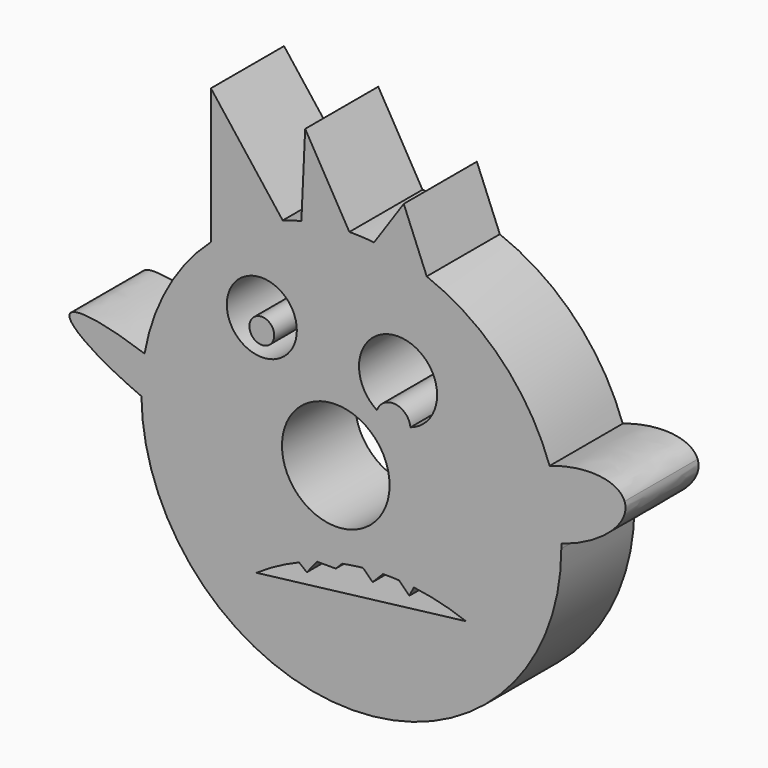
from build123d import *

# Parameters (mm, degrees)
F0_R     = 14.9564951484
F0_R_2   = 9.7335574138
F1_DEPTH = 25.4
F0_R_3   = 3.456724349


# Not quite as in the source:
# - a feature names something its author has since deleted; it is built from what else it names
# - the program builds the solid bodies; features that only make, move or delete a surface that nothing else refers to are left out


with BuildPart() as f1:
    # F0 (on Front) → F1 (new body)
    with BuildSketch(Plane.XZ):
        with BuildLine():
            Line((29.2069212967, 44.8178982187), (-33.0534157144, 44.8178982187))
            ThreePointArc((-33.0534157144, 44.8178982187), (-33.8848589906, 44.1111281894), (-34.7029421619, 43.3889358876))
            ThreePointArc((-34.7029421619, 43.3889358876), (-46.7244943553, 28.2782026704), (-53.157396148, 10.0718919506))
            add(Edge.make_bspline(
                [(-54.0295326022, -0.6419861495), (-25.6291677814, -12.7776607333), (-25.1074200255, -6.368179936), (-24.5856722696, 0.0413008612), (-53.157396148, 10.0718919506)],
                knots=[1.4674967071, 1.4674967071, 1.4674967071, 3.2032565901, 3.2032565901, 4.9390164731, 4.9390164731, 4.9390164731], degree=2, weights=[1, 0.646445519, 1, 0.646445519, 1]))
            ThreePointArc((-54.0295326022, -0.6419861495), (4.6490094653, -58.3601924627), (62.6890867818, 0))
            ThreePointArc((62.6890867818, 0), (62.6859343797, 0.6065848839), (62.6764775138, 1.2131042379))
            add(Edge.make_bspline(
                [(59.4330403873, 19.2211055653), (41.4698148053, 12.9716188145), (43.0336953944, 4.2887424007), (44.5975759835, -4.3941340131), (62.6764775138, 1.2131042379)],
                knots=[1.5260344916, 1.5260344916, 1.5260344916, 3.0598387567, 3.0598387567, 4.5936430218, 4.5936430218, 4.5936430218], degree=2, weights=[1, 0.720063756, 1, 0.720063756, 1]))
            ThreePointArc((59.4330403873, 19.2211055653), (46.2413654037, 40.611400757), (25.2778493531, 54.4712713212))
            Line((25.2778493531, 54.4712713212), (29.2069212967, 44.8178982187))
        make_face()
        Circle(F0_R, mode=Mode.SUBTRACT)
        with BuildLine():
            ThreePointArc((21.6792569731, -22.7834417511), (29.0444233173, -24.1430496826), (36.1979231238, -26.361528784))
            Line((36.1979231238, -26.361528784), (-22.0335181803, -33.4437340498))
            ThreePointArc((-22.0335181803, -33.4437340498), (-16.2921483285, -29.9333256583), (-10.2111068854, -27.0510991203))
            Line((-10.2111068854, -27.0510991204), (-14.6030960605, -23.5375072807))
            Line((-14.6030960605, -23.5375072807), (5.047085695, -20.1314762235))
            Line((5.047085695, -20.1314762235), (24.1732671857, -17.7734531462))
            Line((24.1732671857, -17.7734531462), (21.6792569731, -22.7834417511))
        make_face(mode=Mode.SUBTRACT)
        with Locations((-20.5633433886, 29.5139586047)):
            Circle(F0_R_2, mode=Mode.SUBTRACT)
        with BuildLine():
            ThreePointArc((11.440167814, 17.2330375959), (12.1122768861, 35.8889061597), (28.1660100748, 26.361534372))
            ThreePointArc((28.1660100748, 26.361534372), (26.117377722, 20.0153029261), (20.7448195069, 16.0647122986))
            ThreePointArc((20.7448195069, 16.0647122986), (20.7622755027, 15.8287118822), (20.7680988698, 15.5921384334))
            ThreePointArc((20.7680988698, 15.5921384334), (15.1267587025, 10.8565590643), (11.440167814, 17.2330375959))
        make_face(mode=Mode.SUBTRACT)
        with BuildLine():
            ThreePointArc((-14.7525066988, 55.1538659378), (-24.3720908883, 50.8165251157), (-33.0534157144, 44.8178982187))
            Line((-33.0534157144, 44.8178982187), (29.2069212967, 44.8178982187))
            Line((29.2069212967, 44.8178982187), (25.2778493531, 54.4712713212))
            ThreePointArc((25.2778493531, 54.4712713212), (18.0685855983, 56.7204701), (10.6292413524, 58.0199069867))
            Line((10.6292413524, 58.0199069867), (7.0293885895, 52.7346457751))
            Line((7.0293885895, 52.7346457751), (3.7755604577, 58.3584604129))
            ThreePointArc((3.7755604577, 58.3584604129), (-2.9439825789, 57.9062449617), (-9.5666869161, 56.6829115246))
            Line((-9.5666869161, 56.6829115246), (-9.9255512055, 48.9001048884))
            Line((-9.9255512055, 48.9001048884), (-14.7525066988, 55.1538659378))
        make_face()
        with BuildLine():
            ThreePointArc((-34.7029421619, 43.3889358876), (-33.8848589906, 44.1111281894), (-33.0534157144, 44.8178982187))
            ThreePointArc((-33.0534157144, 44.8178982187), (-24.3720908883, 50.8165251157), (-14.7525066988, 55.1538659378))
            Line((-14.7525066988, 55.1538659378), (-34.7029421619, 81.0014745162))
            Line((-34.7029421619, 81.0014745162), (-34.7029421619, 43.3889358876))
        make_face()
        with BuildLine():
            add(Edge.make_bspline(
                [(80.264955759, 17.3160471022), (77.2571204557, 25.4221829679), (59.4330403873, 19.2211055653)],
                knots=[0, 0, 0, 1.5260344916, 1.5260344916, 1.5260344916], degree=2, weights=[1, 0.7227540692, 1]))
            ThreePointArc((59.4330403873, 19.2211055653), (61.7648977694, 10.3450086355), (62.6764775138, 1.2131042379))
            add(Edge.make_bspline(
                [(62.6764775138, 1.2131042379), (83.8081315933, 7.7671649955), (80.264955759, 17.3160471022)],
                knots=[4.5936430218, 4.5936430218, 4.5936430218, 6.2831853072, 6.2831853072, 6.2831853072], degree=2, weights=[1, 0.6639024438, 1]))
        make_face()
        with BuildLine():
            ThreePointArc((62.6764775138, 1.2131042379), (61.7648977694, 10.3450086355), (59.4330403873, 19.2211055653))
            add(Edge.make_bspline(
                [(59.4330403873, 19.2211055653), (41.4698148053, 12.9716188145), (43.0336953944, 4.2887424007), (44.5975759835, -4.3941340131), (62.6764775138, 1.2131042379)],
                knots=[1.5260344916, 1.5260344916, 1.5260344916, 3.0598387567, 3.0598387567, 4.5936430218, 4.5936430218, 4.5936430218], degree=2, weights=[1, 0.720063756, 1, 0.720063756, 1]))
        make_face()
        with BuildLine():
            add(Edge.make_bspline(
                [(-54.0295326022, -0.6419861495), (-25.6291677814, -12.7776607333), (-25.1074200255, -6.368179936), (-24.5856722696, 0.0413008612), (-53.157396148, 10.0718919506)],
                knots=[1.4674967071, 1.4674967071, 1.4674967071, 3.2032565901, 3.2032565901, 4.9390164731, 4.9390164731, 4.9390164731], degree=2, weights=[1, 0.646445519, 1, 0.646445519, 1]))
            ThreePointArc((-53.157396148, 10.0718919506), (-53.840658448, 4.7350751159), (-54.0295326022, -0.6419861495))
        make_face()
        with BuildLine():
            ThreePointArc((-54.0295326022, -0.6419861495), (-53.840658448, 4.7350751159), (-53.157396148, 10.0718919506))
            add(Edge.make_bspline(
                [(-53.157396148, 10.0718919506), (-72.4188899566, 16.8339679453), (-73.9696696401, 12.9880346358)],
                knots=[4.9390164731, 4.9390164731, 4.9390164731, 6.2831853072, 6.2831853072, 6.2831853072], degree=2, weights=[1, 0.7825255703, 1]))
            add(Edge.make_bspline(
                [(-73.9696696401, 12.9880346358), (-75.7271245891, 8.6295467082), (-54.0295326022, -0.6419861495)],
                knots=[0, 0, 0, 1.4674967071, 1.4674967071, 1.4674967071], degree=2, weights=[1, 0.7426695101, 1]))
        make_face()
        with BuildLine():
            Line((-8.5103068977, 79.5929687748), (-9.5666869161, 56.6829115246))
            ThreePointArc((-9.5666869161, 56.6829115246), (-2.9439825789, 57.9062449617), (3.7755604577, 58.3584604129))
            Line((3.7755604577, 58.3584604129), (-8.5103068977, 79.5929687748))
        make_face()
        with BuildLine():
            ThreePointArc((10.6292413524, 58.0199069867), (18.0685855983, 56.7204701), (25.2778493531, 54.4712713212))
            Line((25.2778493531, 54.4712713212), (18.8944284965, 70.1547569089))
            Line((18.8944284965, 70.1547569089), (10.6292413524, 58.0199069867))
        make_face()
        with BuildLine():
            ThreePointArc((17.581953772, -22.4095073895), (19.6336387932, -22.5632365329), (21.6792569731, -22.7834417511))
            Line((21.6792569731, -22.7834417511), (24.1732671857, -17.7734531462))
            Line((24.1732671857, -17.7734531462), (5.047085695, -20.1314762235))
            Line((5.047085695, -20.1314762235), (7.5632852876, -22.6151940263))
            ThreePointArc((7.5632852876, -22.6151940263), (10.3425062964, -22.398982827), (13.1285441555, -22.3051225785))
            Line((13.1285441555, -22.3051225785), (15.2741307635, -20.1314762235))
            Line((15.2741307635, -20.1314762235), (17.581953772, -22.4095073895))
        make_face()
        with BuildLine():
            Line((-14.6030960605, -23.5375072807), (-10.2111068854, -27.0510991204))
            ThreePointArc((-10.2111068854, -27.0510991203), (-7.7377628762, -26.0957196312), (-5.2266436009, -25.2445671531))
            ThreePointArc((-5.2266436009, -25.2445671531), (-1.7623985905, -24.2578232608), (1.7522839969, -23.4693669777))
            Line((1.7522839969, -23.4693669777), (5.047085695, -20.1314762235))
            Line((5.047085695, -20.1314762235), (-14.6030960605, -23.5375072807))
        make_face()
        with BuildLine():
            ThreePointArc((20.7448195069, 16.0647122986), (15.9598060497, 15.5921384334), (11.440167814, 17.2330375959))
            ThreePointArc((11.440167814, 17.2330375959), (15.1267587025, 10.8565590643), (20.7680988698, 15.5921384334))
            ThreePointArc((20.7680988698, 15.5921384334), (20.7622755027, 15.8287118822), (20.7448195069, 16.0647122986))
        make_face()
        with BuildLine():
            ThreePointArc((20.7448195069, 16.0647122986), (16.5588486209, 20.3629693716), (11.440167814, 17.2330375959))
            ThreePointArc((11.440167814, 17.2330375959), (15.9598060497, 15.5921384334), (20.7448195069, 16.0647122986))
        make_face()
        with BuildLine():
            ThreePointArc((-9.5666869161, 56.6829115246), (-12.1773125744, 55.9784724693), (-14.7525066988, 55.1538659378))
            Line((-14.7525066988, 55.1538659378), (-9.9255512055, 48.9001048884))
            Line((-9.9255512055, 48.9001048884), (-9.5666869161, 56.6829115246))
        make_face()
        with BuildLine():
            ThreePointArc((10.6292413524, 58.0199069867), (7.2073810591, 58.2900020166), (3.7755604577, 58.3584604129))
            Line((3.7755604577, 58.3584604129), (7.0293885895, 52.7346457751))
            Line((7.0293885895, 52.7346457751), (10.6292413524, 58.0199069867))
        make_face()
        with BuildLine():
            Line((7.5632852876, -22.6151940263), (5.047085695, -20.1314762235))
            Line((5.047085695, -20.1314762235), (1.7522839969, -23.4693669777))
            ThreePointArc((1.7522839969, -23.4693669777), (4.6478901063, -22.9749672477), (7.5632852876, -22.6151940263))
        make_face()
        with BuildLine():
            Line((10.2270450686, -25.2445671531), (13.1285441555, -22.3051225785))
            ThreePointArc((13.1285441555, -22.3051225785), (10.3425062964, -22.398982827), (7.5632852876, -22.6151940263))
            Line((7.5632852876, -22.6151940263), (10.2270450686, -25.2445671531))
        make_face()
        with BuildLine():
            ThreePointArc((-5.2266436009, -25.2445671531), (-7.7377628762, -26.0957196312), (-10.2111068854, -27.0510991203))
            Line((-10.2111068854, -27.0510991204), (-8.0530354753, -28.7775564939))
            Line((-8.0530354753, -28.7775564939), (-5.2266436009, -25.2445671531))
        make_face()
        with BuildLine():
            Line((20.4540901372, -25.2445671531), (21.6792569731, -22.7834417511))
            ThreePointArc((21.6792569731, -22.7834417511), (19.6336387932, -22.5632365329), (17.581953772, -22.4095073895))
            Line((17.581953772, -22.4095073895), (20.4540901372, -25.2445671531))
        make_face()
        with BuildLine():
            ThreePointArc((1.7522839969, -23.4693669777), (-1.7623985905, -24.2578232608), (-5.2266436009, -25.2445671531))
            Line((-5.2266436009, -25.2445671531), (0, -25.2445671531))
            Line((0, -25.2445671531), (1.7522839969, -23.4693669777))
        make_face()
        with BuildLine():
            ThreePointArc((13.1285441555, -22.3051225785), (15.356165832, -22.3181982774), (17.581953772, -22.4095073895))
            Line((17.581953772, -22.4095073895), (15.2741307635, -20.1314762235))
            Line((15.2741307635, -20.1314762235), (13.1285441555, -22.3051225785))
        make_face()
    extrude(amount=F1_DEPTH)


with BuildPart() as f1b:
    # F0 (on Front) → F1, piece 2 (new body)
    with BuildSketch(Plane.XZ):
        with Locations((-20.5633433886, 26.2429621071)):
            Circle(F0_R_3)
    extrude(amount=F1_DEPTH)


solid = Compound([f1.part, f1b.part])
